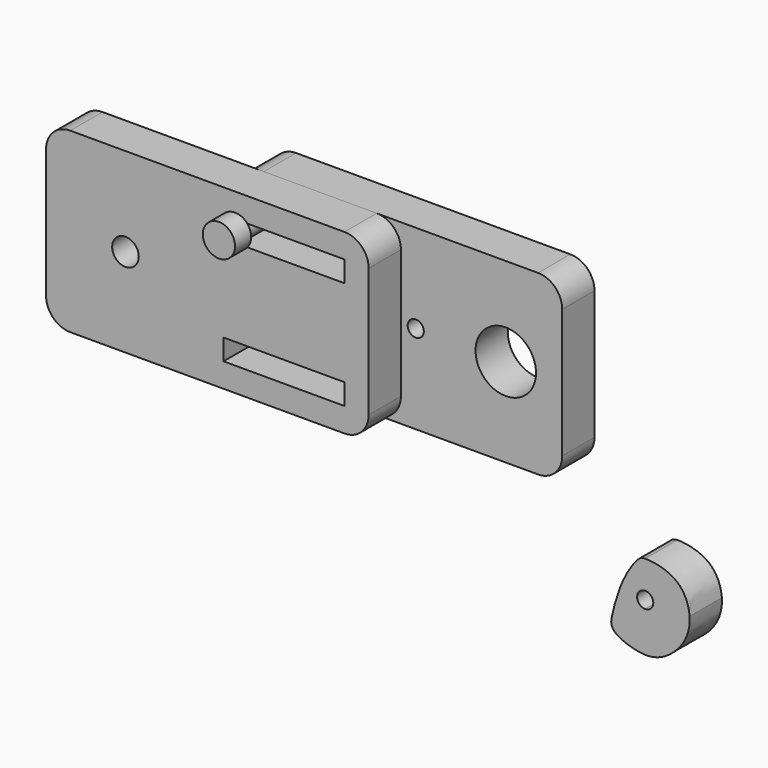
from build123d import *

# Parameters (mm, degrees)
F0_R      = 4.191
F1_DEPTH  = 12.7
F2_R      = 2.54
F3_DEPTH  = 12.7
F5_DEPTH  = 12.7
F7_DEPTH  = 25.4
F8_R      = 5.08
F9_DEPTH  = 6.35
F11_R     = 5.08
F12_DEPTH = 6.35


# Not quite as in the source:
# - a feature names something its author has since deleted; it is built from what else it names


with BuildPart() as f1:
    # F0 (on Front) → F1 (new body)
    with BuildSketch(Plane.XZ):
        with BuildLine():
            Line((-139.9206458214, 96.2469654174), (-147.5546886596, 96.2469654174))
            ThreePointArc((-147.5546886596, 96.2469654174), (-152.9428423322, 94.01511909), (-155.1746886596, 88.6269654174))
            Line((-155.1746886596, 88.6269654174), (-155.1746886596, 84.1381776578))
            ThreePointArc((-155.1746886596, 84.1381776578), (-148.5724078124, 91.4834882579), (-139.9206458214, 96.2469654174))
        make_face()
        with BuildLine():
            Line((-120.4287314978, 96.2469654174), (-139.9206458214, 96.2469654174))
            ThreePointArc((-139.9206458214, 96.2469654174), (-148.5724078124, 91.4834882579), (-155.1746886596, 84.1381776578))
            Line((-155.1746886596, 84.1381776578), (-155.1746886596, 52.475753177))
            ThreePointArc((-155.1746886596, 52.475753177), (-148.5724078124, 45.1304425769), (-139.9206458214, 40.3669654174))
            Line((-139.9206458214, 40.3669654174), (-120.4287314978, 40.3669654174))
            ThreePointArc((-120.4287314978, 40.3669654174), (-106.0498062829, 51.1716996969), (-100.5836886596, 68.3069654174))
            ThreePointArc((-100.5836886596, 68.3069654174), (-106.0498062829, 85.4422311379), (-120.4287314978, 96.2469654174))
        make_face()
        with Locations((-130.1746886596, 68.3069654174)):
            Circle(F0_R, mode=Mode.SUBTRACT)
        with BuildLine():
            ThreePointArc((-139.9206458214, 40.3669654174), (-148.5724078124, 45.1304425769), (-155.1746886596, 52.475753177))
            Line((-155.1746886596, 52.475753177), (-155.1746886596, 47.9869654174))
            ThreePointArc((-155.1746886596, 47.9869654174), (-152.9428423322, 42.5988117447), (-147.5546886596, 40.3669654174))
            Line((-147.5546886596, 40.3669654174), (-139.9206458214, 40.3669654174))
        make_face()
        with BuildLine():
            Line((-61.1946886596, 96.2469654174), (-120.4287314978, 96.2469654174))
            ThreePointArc((-120.4287314978, 96.2469654174), (-106.0498062829, 85.4422311379), (-100.5836886596, 68.3069654174))
            ThreePointArc((-100.5836886596, 68.3069654174), (-106.0498062829, 51.1716996969), (-120.4287314978, 40.3669654174))
            Line((-120.4287314978, 40.3669654174), (-61.1946886596, 40.3669654174))
            ThreePointArc((-61.1946886596, 40.3669654174), (-55.806534987, 42.5988117447), (-53.5746886596, 47.9869654174))
            Line((-53.5746886596, 47.9869654174), (-53.5746886596, 63.2269654174))
            ThreePointArc((-53.5746886596, 63.2269654174), (-53.885666586, 65.7585092834), (-53.9895557072, 68.3069654174))
            ThreePointArc((-53.9895557072, 68.3069654174), (-53.885666586, 70.8554215514), (-53.5746886596, 73.3869654174))
            Line((-53.5746886596, 73.3869654174), (-53.5746886596, 88.6269654174))
            ThreePointArc((-53.5746886596, 88.6269654174), (-55.806534987, 94.01511909), (-61.1946886596, 96.2469654174))
        make_face()
        with BuildLine():
            Line((-61.1946886596, 47.9869654174), (-99.2946886596, 47.9869654174))
            ThreePointArc((-99.2946886596, 47.9869654174), (-102.5966886596, 51.2889654174), (-99.2946886596, 54.5909654174))
            Line((-99.2946886596, 54.5909654174), (-61.1946886596, 54.5909654174))
            ThreePointArc((-61.1946886596, 54.5909654174), (-57.8926886596, 51.2889654174), (-61.1946886596, 47.9869654174))
        make_face(mode=Mode.SUBTRACT)
        with BuildLine():
            ThreePointArc((-99.2946886596, 82.0229654174), (-102.5966886596, 85.3249654174), (-99.2946886596, 88.6269654174))
            Line((-99.2946886596, 88.6269654174), (-61.1946886596, 88.6269654174))
            ThreePointArc((-61.1946886596, 88.6269654174), (-57.8926886596, 85.3249654174), (-61.1946886596, 82.0229654174))
            Line((-61.1946886596, 82.0229654174), (-99.2946886596, 82.0229654174))
        make_face(mode=Mode.SUBTRACT)
        with BuildLine():
            ThreePointArc((-61.1946886596, 82.0229654174), (-57.8926886596, 85.3249654174), (-61.1946886596, 88.6269654174))
            Line((-61.1946886596, 88.6269654174), (-61.1946886596, 82.0229654174))
        make_face()
        with BuildLine():
            Line((-99.2946886596, 82.0229654174), (-99.2946886596, 88.6269654174))
            ThreePointArc((-99.2946886596, 88.6269654174), (-102.5966886596, 85.3249654174), (-99.2946886596, 82.0229654174))
        make_face()
        with BuildLine():
            ThreePointArc((-99.2946886596, 54.5909654174), (-102.5966886596, 51.2889654174), (-99.2946886596, 47.9869654174))
            Line((-99.2946886596, 47.9869654174), (-99.2946886596, 54.5909654174))
        make_face()
        with BuildLine():
            Line((-61.1946886596, 54.5909654174), (-61.1946886596, 47.9869654174))
            ThreePointArc((-61.1946886596, 47.9869654174), (-57.8926886596, 51.2889654174), (-61.1946886596, 54.5909654174))
        make_face()
        with BuildLine():
            Line((-53.5746886596, 63.2269654174), (-53.5746886596, 68.3069654174))
            Line((-53.5746886596, 68.3069654174), (-53.9895557072, 68.3069654174))
            ThreePointArc((-53.9895557072, 68.3069654174), (-53.885666586, 65.7585092834), (-53.5746886596, 63.2269654174))
        make_face()
        with BuildLine():
            Line((-53.5746886596, 68.3069654174), (-53.5746886596, 73.3869654174))
            ThreePointArc((-53.5746886596, 73.3869654174), (-53.885666586, 70.8554215514), (-53.9895557072, 68.3069654174))
            Line((-53.9895557072, 68.3069654174), (-53.5746886596, 68.3069654174))
        make_face()
    extrude(amount=F1_DEPTH)


with BuildPart() as f3:
    # F2 (on face) → F3 (new body)
    with BuildSketch(Plane(origin=(0, 0, 0), x_dir=(-1, 0, 0), z_dir=(0, 1, 0))):
        with BuildLine():
            Line((104.3746886596, 53.816027525), (104.3746886596, 82.7979033097))
            ThreePointArc((104.3746886596, 82.7979033097), (100.5836886596, 68.3069654174), (104.3746886596, 53.816027525))
        make_face()
        with BuildLine():
            ThreePointArc((104.3746886596, 53.816027525), (100.5836886596, 68.3069654174), (104.3746886596, 82.7979033097))
            Line((104.3746886596, 82.7979033097), (104.3746886596, 88.6269654174))
            ThreePointArc((104.3746886596, 88.6269654174), (102.1428423322, 94.01511909), (96.7546886596, 96.2469654174))
            Line((96.7546886596, 96.2469654174), (61.1946886596, 96.2469654174))
            ThreePointArc((61.1946886596, 96.2469654174), (55.806534987, 94.01511909), (53.5746886596, 88.6269654174))
            Line((53.5746886596, 88.6269654174), (53.5746886596, 47.9869654174))
            ThreePointArc((53.5746886596, 47.9869654174), (55.806534987, 42.5988117447), (61.1946886596, 40.3669654174))
            Line((61.1946886596, 40.3669654174), (96.7546886596, 40.3669654174))
            ThreePointArc((96.7546886596, 40.3669654174), (102.1428423322, 42.5988117447), (104.3746886596, 47.9869654174))
            Line((104.3746886596, 47.9869654174), (104.3746886596, 53.816027525))
        make_face()
        with BuildLine():
            Line((98.0246886596, 47.9869654174), (61.1946886596, 47.9869654174))
            ThreePointArc((61.1946886596, 47.9869654174), (57.8926886596, 51.2889654174), (61.1946886596, 54.5909654174))
            Line((61.1946886596, 54.5909654174), (98.0246886596, 54.5909654174))
            Line((98.0246886596, 54.5909654174), (99.2946886596, 54.5909654174))
            Line((99.2946886596, 54.5909654174), (99.2946886596, 54.3369654174))
            ThreePointArc((99.2946886596, 54.3369654174), (101.3266886596, 51.2889654174), (99.2946886596, 48.2409654174))
            Line((99.2946886596, 48.2409654174), (99.2946886596, 47.9869654174))
            Line((99.2946886596, 47.9869654174), (98.0246886596, 47.9869654174))
        make_face(mode=Mode.SUBTRACT)
        with BuildLine():
            ThreePointArc((61.1946886596, 82.0229654174), (57.8926886596, 85.3249654174), (61.1946886596, 88.6269654174))
            Line((61.1946886596, 88.6269654174), (98.0246886596, 88.6269654174))
            Line((98.0246886596, 88.6269654174), (99.2946886596, 88.6269654174))
            Line((99.2946886596, 88.6269654174), (99.2946886596, 88.3729654174))
            ThreePointArc((99.2946886596, 88.3729654174), (101.3266886596, 85.3249654174), (99.2946886596, 82.2769654174))
            Line((99.2946886596, 82.2769654174), (99.2946886596, 82.0229654174))
            Line((99.2946886596, 82.0229654174), (98.0246886596, 82.0229654174))
            Line((98.0246886596, 82.0229654174), (61.1946886596, 82.0229654174))
        make_face(mode=Mode.SUBTRACT)
        with BuildLine():
            ThreePointArc((53.5746886596, 88.6269654174), (55.806534987, 94.01511909), (61.1946886596, 96.2469654174))
            Line((61.1946886596, 96.2469654174), (10.3946886596, 96.2469654174))
            ThreePointArc((10.3946886596, 96.2469654174), (5.006534987, 94.01511909), (2.7746886596, 88.6269654174))
            Line((2.7746886596, 88.6269654174), (2.7746886596, 68.3069654174))
            Line((2.7746886596, 68.3069654174), (2.7746886596, 47.9869654174))
            ThreePointArc((2.7746886596, 47.9869654174), (5.006534987, 42.5988117447), (10.3946886596, 40.3669654174))
            Line((10.3946886596, 40.3669654174), (61.1946886596, 40.3669654174))
            ThreePointArc((61.1946886596, 40.3669654174), (55.806534987, 42.5988117447), (53.5746886596, 47.9869654174))
            Line((53.5746886596, 47.9869654174), (53.5746886596, 88.6269654174))
        make_face()
        with BuildLine():
            ThreePointArc((30.0796886596, 68.3069654174), (20.5546886596, 58.7819654174), (11.0296886596, 68.3069654174))
            ThreePointArc((11.0296886596, 68.3069654174), (20.5546886596, 77.8319654174), (30.0796886596, 68.3069654174))
        make_face(mode=Mode.SUBTRACT)
        with Locations((48.9087601889, 68.3069654174)):
            Circle(F2_R, mode=Mode.SUBTRACT)
        with BuildLine():
            Line((61.1946886596, 82.0229654174), (61.1946886596, 88.6269654174))
            ThreePointArc((61.1946886596, 88.6269654174), (57.8926886596, 85.3249654174), (61.1946886596, 82.0229654174))
        make_face()
        with BuildLine():
            ThreePointArc((99.2946886596, 82.2769654174), (101.3266886596, 85.3249654174), (99.2946886596, 88.3729654174))
            Line((99.2946886596, 88.3729654174), (99.2946886596, 82.2769654174))
        make_face()
        with BuildLine():
            ThreePointArc((61.1946886596, 54.5909654174), (57.8926886596, 51.2889654174), (61.1946886596, 47.9869654174))
            Line((61.1946886596, 47.9869654174), (61.1946886596, 54.5909654174))
        make_face()
        with BuildLine():
            Line((99.2946886596, 54.3369654174), (99.2946886596, 48.2409654174))
            ThreePointArc((99.2946886596, 48.2409654174), (101.3266886596, 51.2889654174), (99.2946886596, 54.3369654174))
        make_face()
    extrude(amount=F3_DEPTH)


with BuildPart() as f5:
    # F4 (on face) → F5 (new body)
    with BuildSketch(Plane.XZ):
        with BuildLine():
            Line((-34.9387601889, 68.3069654174), (-46.3687601889, 68.3069654174))
            ThreePointArc((-46.3687601889, 68.3069654174), (-47.1127089646, 66.5109141932), (-48.9087601889, 65.7669654174))
            Line((-48.9087601889, 65.7669654174), (-48.9087601889, 53.0669654174))
            add(Edge.make_bspline(
                [(-48.9087601889, 53.0669654174), (-46.3285467286, 52.9238934617), (-41.4799378473, 54.7230419503), (-35.8287521803, 60.8381500164), (-34.7770086547, 65.8512725443), (-34.9387601889, 68.3069654174)],
                knots=[0.2340557088, 0.2340557088, 0.2340557088, 0.2340557088, 0.3646239146, 0.5002137772, 0.6297444601, 0.6297444601, 0.6297444601, 0.6297444601], degree=3))
        make_face()
        with BuildLine():
            Line((-48.9087601889, 79.7369654174), (-48.9087601889, 70.8469654174))
            ThreePointArc((-48.9087601889, 70.8469654174), (-47.1127089646, 70.1030166416), (-46.3687601889, 68.3069654174))
            Line((-46.3687601889, 68.3069654174), (-34.9387601889, 68.3069654174))
            add(Edge.make_bspline(
                [(-34.9387601889, 68.3069654174), (-35.0983756624, 70.7302288685), (-36.6987277791, 75.4863182563), (-42.6519902081, 79.0895832696), (-46.7267623422, 79.7235088874), (-48.9087601889, 79.7369654174)],
                knots=[0.6297444601, 0.6297444601, 0.6297444601, 0.6297444601, 0.7575645849, 0.8799690979, 1, 1, 1, 1], degree=3))
        make_face()
        with BuildLine():
            ThreePointArc((-48.9087601889, 65.7669654174), (-51.4487601889, 68.3069654174), (-48.9087601889, 70.8469654174))
            Line((-48.9087601889, 70.8469654174), (-48.9087601889, 79.7369654174))
            add(Edge.make_bspline(
                [(-48.9087601889, 79.7369654174), (-49.649387598, 79.7235088874), (-52.0489108643, 79.6773670628), (-52.2937670227, 68.2091246166), (-56.8141028195, 60.6082690604), (-59.1832799759, 60.1315936113), (-59.8948027841, 58.4826101727), (-59.1975102164, 57.5251552323), (-58.8302104007, 57.0208143578)],
                knots=[0, 0, 0, 0, 0.1258899192, 0.4080535306, 0.6632334705, 0.784728135, 0.8866053092, 1, 1, 1, 1], degree=3))
            add(Edge.make_bspline(
                [(-58.8302104007, 57.0208143578), (-58.1551886307, 56.5514570937), (-55.7954730291, 55.0381703125), (-51.5908464478, 53.2156861849), (-48.9087601889, 53.0669654174)],
                knots=[0.0372724804, 0.0372724804, 0.0372724804, 0.0372724804, 0.0983323681, 0.2340557088, 0.2340557088, 0.2340557088, 0.2340557088], degree=3))
            Line((-48.9087601889, 53.0669654174), (-48.9087601889, 65.7669654174))
        make_face()
    extrude(amount=F5_DEPTH)


with BuildPart() as f5b:
    # F4 (on face) → F5, piece 2 (new body)
    with BuildSketch(Plane.XZ):
        with BuildLine():
            ThreePointArc((33.5207186108, 22.4936557771), (30.9807186108, 25.0336557771), (33.5207186108, 27.5736557771))
            Line((33.5207186108, 27.5736557771), (33.5207186108, 36.4636557771))
            add(Edge.make_bspline(
                [(33.5207186108, 9.7936557771), (30.5818251845, 9.8753367916), (25.1895329136, 11.650086509), (23.151634381, 13.7747889217), (22.6297846964, 15.3984872991), (23.3899658492, 19.1000192408), (25.6937335032, 26.8787970737), (28.5310883181, 32.0844700515), (31.3367132034, 35.9862495236), (32.6430004787, 36.4281003314), (33.5207186108, 36.4636557771)],
                knots=[0.4902707627, 0.4902707627, 0.4902707627, 0.4902707627, 0.5804219713, 0.6306678411, 0.6674243671, 0.7256146555, 0.813759797, 0.8909140141, 0.9552136893, 1, 1, 1, 1], degree=3))
            Line((33.5207186108, 9.7936557771), (33.5207186108, 22.4936557771))
        make_face()
        with BuildLine():
            Line((47.4907186108, 25.0336557771), (36.0607186108, 25.0336557771))
            ThreePointArc((36.0607186108, 25.0336557771), (35.316769835, 23.2376045529), (33.5207186108, 22.4936557771))
            Line((33.5207186108, 22.4936557771), (33.5207186108, 9.7936557771))
            add(Edge.make_bspline(
                [(47.4907186108, 25.0336557771), (47.6697702401, 22.5776243447), (46.6116425624, 17.5740579937), (40.8817647302, 11.4169450372), (36.2452293961, 9.7179331249), (33.5207186108, 9.7936557771)],
                knots=[0.236995651, 0.236995651, 0.236995651, 0.236995651, 0.3199065199, 0.4066957892, 0.4902707627, 0.4902707627, 0.4902707627, 0.4902707627], degree=3))
        make_face()
        with BuildLine():
            Line((33.5207186108, 36.4636557771), (33.5207186108, 27.5736557771))
            ThreePointArc((33.5207186108, 27.5736557771), (35.316769835, 26.8297070013), (36.0607186108, 25.0336557771))
            Line((36.0607186108, 25.0336557771), (47.4907186108, 25.0336557771))
            add(Edge.make_bspline(
                [(33.5207186108, 36.4636557771), (35.0264297479, 36.5246505642), (40.096951526, 35.7809150246), (45.6413349227, 32.2235422638), (47.3140315038, 27.4572533167), (47.4907186108, 25.0336557771)],
                knots=[0, 0, 0, 0, 0.0768301854, 0.1551796877, 0.236995651, 0.236995651, 0.236995651, 0.236995651], degree=3))
        make_face()
    extrude(amount=F5_DEPTH)


with BuildPart() as f7:
    # F6 (on face) → F7 (new body)
    with BuildSketch(Plane.XZ.offset(12.7)):
        with BuildLine():
            Line((-98.8628707164, 86.1419352524), (-98.8628707164, 84.5079955824))
            ThreePointArc((-98.8628707164, 84.5079955824), (-92.3615326147, 85.3249654174), (-98.8628707164, 86.1419352524))
        make_face()
    extrude(amount=-F7_DEPTH)

    # F8 (on face) → F9 (join)
    with BuildSketch(Plane.XZ.offset(12.7)):
        with Locations((-95.6635326147, 85.3249654174)):
            Circle(F8_R)
    extrude(amount=F9_DEPTH)

    # F11 (on face) → F12 (join)
    with BuildSketch(Plane(origin=(0, 12.7, 0), x_dir=(-1, 0, 0), z_dir=(0, 1, 0))):
        with Locations((95.6635326147, 85.3249654174)):
            Circle(F11_R)
    extrude(amount=F12_DEPTH)


solid = Compound([f1.part, f3.part, f5b.part, f7.part])
